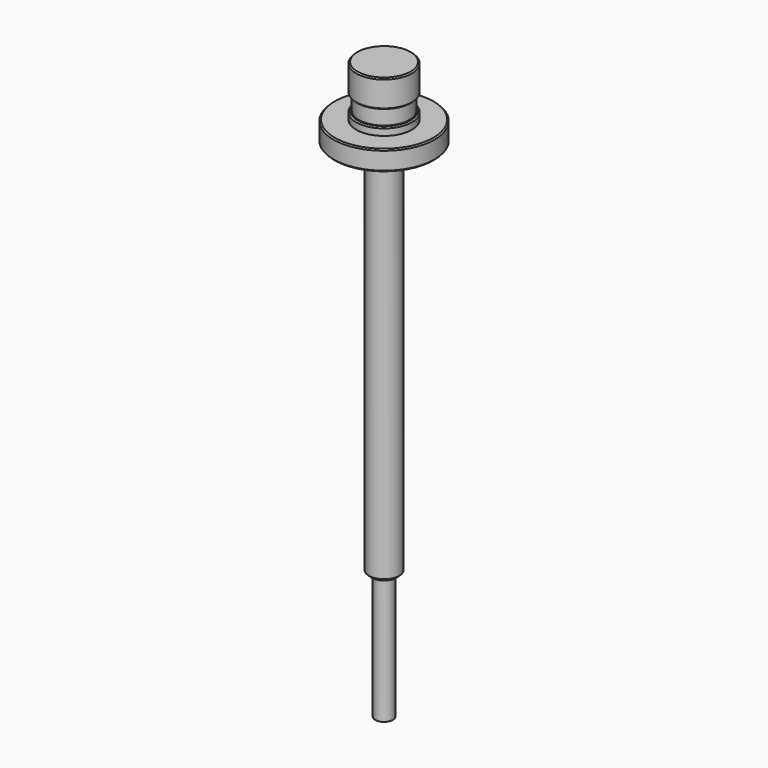
from build123d import *

# Parameters (mm, degrees)
F0_R      = 3.5
F1_DEPTH  = 50
F2_R      = 6
F3_DEPTH  = 150
F4_R      = 20
F5_DEPTH  = 7.9
F6_SIZE   = 1
F7_SIZE   = 0.5
F8_R      = 11
F9_DEPTH  = 3.1
F10_R     = 10
F11_DEPTH = 6
F12_R     = 11
F13_DEPTH = 11
F14_SIZE  = 0.5


with BuildPart() as f1:
    # F0 (on Top) → F1 (new body)
    with BuildSketch(Plane.XY):
        Circle(F0_R)
    extrude(amount=F1_DEPTH)

    # F2 (on face) → F3 (join)
    with BuildSketch(Plane.XY.offset(50)):
        Circle(F2_R)
    extrude(amount=F3_DEPTH)

    # F4 (on face) → F5 (join)
    with BuildSketch(Plane.XY.offset(200)):
        Circle(F4_R)
    extrude(amount=F5_DEPTH)

    # F6
    f6_edges = [f1.edges().sort_by_distance(p)[0] for p in [
        (-6, 0, 50),
    ]]
    chamfer(f6_edges, length=F6_SIZE)

    # F7
    f7_edges = [f1.edges().sort_by_distance(p)[0] for p in [
        (-20, 0, 200),
        (-20, 0, 207.9),
    ]]
    chamfer(f7_edges, length=F7_SIZE)

    # F8 (on face) → F9 (join)
    with BuildSketch(Plane.XY.offset(207.9)):
        Circle(F8_R)
    extrude(amount=F9_DEPTH)

    # F10 (on face) → F11 (join)
    with BuildSketch(Plane.XY.offset(211)):
        Circle(F10_R)
    extrude(amount=F11_DEPTH)

    # F12 (on face) → F13 (join)
    with BuildSketch(Plane.XY.offset(217)):
        Circle(F12_R)
    extrude(amount=F13_DEPTH)

    # F14
    f14_edges = [f1.edges().sort_by_distance(p)[0] for p in [
        (-11, 0, 211),
        (-11, 0, 217),
        (-11, 0, 228),
    ]]
    chamfer(f14_edges, length=F14_SIZE)


solid = f1.part
